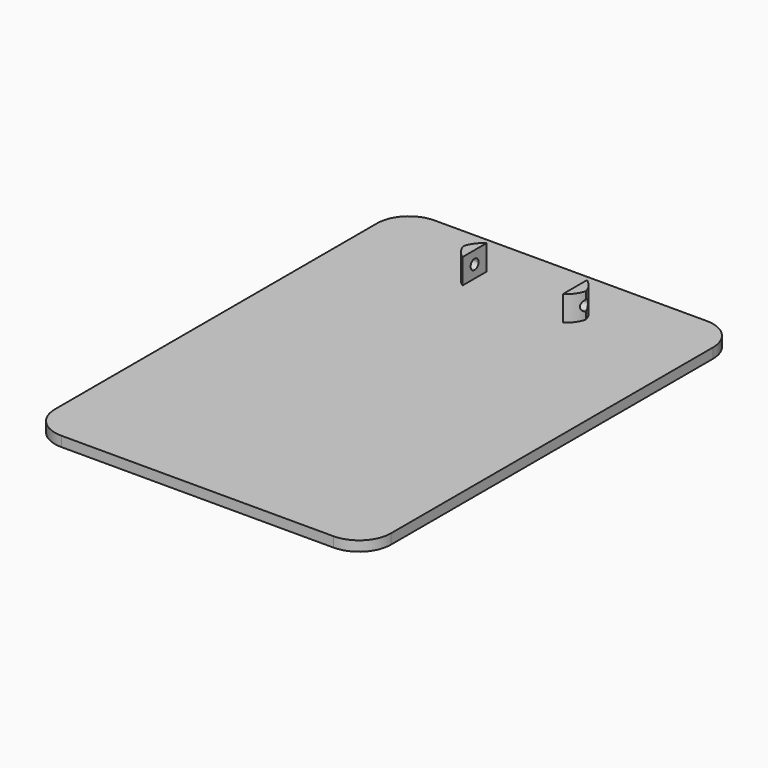
from build123d import *

# Parameters (mm, degrees)
F1_DEPTH    = 2
F3_DEPTH    = 5
F6_DEPTH    = 25.4
F7_T1_DEPTH = 15.711756993


# Not quite as in the source:
# - a fillet or chamfer that OpenCascade refuses, or shapes differently, is made with other operations: its cross-section is extruded or revolved along the edge and cut away or added


with BuildPart() as f1:
    # F0 (on Top) → F1 (new body)
    with BuildSketch(Plane.XY):
        with BuildLine():
            Line((27.15, 46.5), (-27.15, 46.5))
            ThreePointArc((-27.15, 46.5), (-31.6401280605, 44.6401280605), (-33.5, 40.15))
            Line((-33.5, 40.15), (-33.5, -40.15))
            ThreePointArc((-33.5, -40.15), (-31.6401280605, -44.6401280605), (-27.15, -46.5))
            Line((-27.15, -46.5), (27.15, -46.5))
            ThreePointArc((27.15, -46.5), (31.6401280605, -44.6401280605), (33.5, -40.15))
            Line((33.5, -40.15), (33.5, 40.15))
            ThreePointArc((33.5, 40.15), (31.6401280605, 44.6401280605), (27.15, 46.5))
        make_face()
    extrude(amount=F1_DEPTH)

    # F2 (on face) → F3 (join)
    with BuildSketch(Plane.XY.offset(2)):
        Polygon((-11.4712007344, 35.0872650743), (-10, 35.0872650743), (-10, 38.0872650743), (-12.3509485275, 38.0872650743), (-12.3509485275, 35.0872650743), align=None)
        Polygon((-10, 32.0872650743), (-10, 35.0872650743), (-11.4712007344, 35.0872650743), (-12.3509485275, 35.0872650743), (-12.3509485275, 32.0872650743), align=None)
        Polygon((10, 38.0872650743), (10, 35.0872650743), (10, 32.0872650743), (12.3509485275, 32.0872650743), (12.3509485275, 35.0872650743), (12.3509485275, 38.0872650743), align=None)
    extrude(amount=F3_DEPTH)

    # F5 (on face) + F4 (on face) → F6 (cut)
    with BuildSketch(Plane.YZ.offset(12.3509485275)):
        with BuildLine():
            ThreePointArc((36.0872650743, 4.5), (34.3801582931, 5.2071067812), (35.0872650743, 3.5))
            ThreePointArc((35.0872650743, 3.5), (35.7943718554, 3.7928932188), (36.0872650743, 4.5))
        make_face()
    with BuildSketch(Plane(origin=(-12.3509485275, 0, 0), x_dir=(0, -1, 0), z_dir=(-1, 0, 0))):
        with BuildLine():
            ThreePointArc((-34.0872650743, 4.5), (-35.7943718554, 5.2071067812), (-35.0872650743, 3.5))
            ThreePointArc((-35.0872650743, 3.5), (-34.3801582931, 3.7928932188), (-34.0872650743, 4.5))
        make_face()
    extrude(amount=-F6_DEPTH, dir=(1, 0, 0), mode=Mode.SUBTRACT)

    # F7: fillet of radius 5.08 on 4 edges, made by hand

    # F7_s2 → F7_t1 (cut)
    with BuildSketch(Plane.XY.offset(2)):
        with BuildLine():
            ThreePointArc((-12.3509485275, 36.3719678714), (-11.7245976762, 33.9283211581), (-10, 32.0872650743))
            Line((-10, 32.0872650743), (-12.3509485275, 32.0872650743))
            Line((-12.3509485275, 32.0872650743), (-12.3509485275, 36.3719678714))
        make_face()
        with BuildLine():
            ThreePointArc((-10, 38.0872650743), (-11.7245976762, 36.2462089904), (-12.3509485275, 33.8025622771))
            Line((-12.3509485275, 33.8025622771), (-12.3509485275, 38.0872650743))
            Line((-12.3509485275, 38.0872650743), (-10, 38.0872650743))
        make_face()
        with BuildLine():
            ThreePointArc((10, 32.0872650743), (11.7245976762, 33.9283211581), (12.3509485275, 36.3719678714))
            Line((12.3509485275, 36.3719678714), (12.3509485275, 32.0872650743))
            Line((12.3509485275, 32.0872650743), (10, 32.0872650743))
        make_face()
        with BuildLine():
            ThreePointArc((10, 38.0872650743), (11.7245976762, 36.2462089904), (12.3509485275, 33.8025622771))
            Line((12.3509485275, 33.8025622771), (12.3509485275, 38.0872650743))
            Line((12.3509485275, 38.0872650743), (10, 38.0872650743))
        make_face()
    extrude(amount=F7_T1_DEPTH, mode=Mode.SUBTRACT)


solid = f1.part
